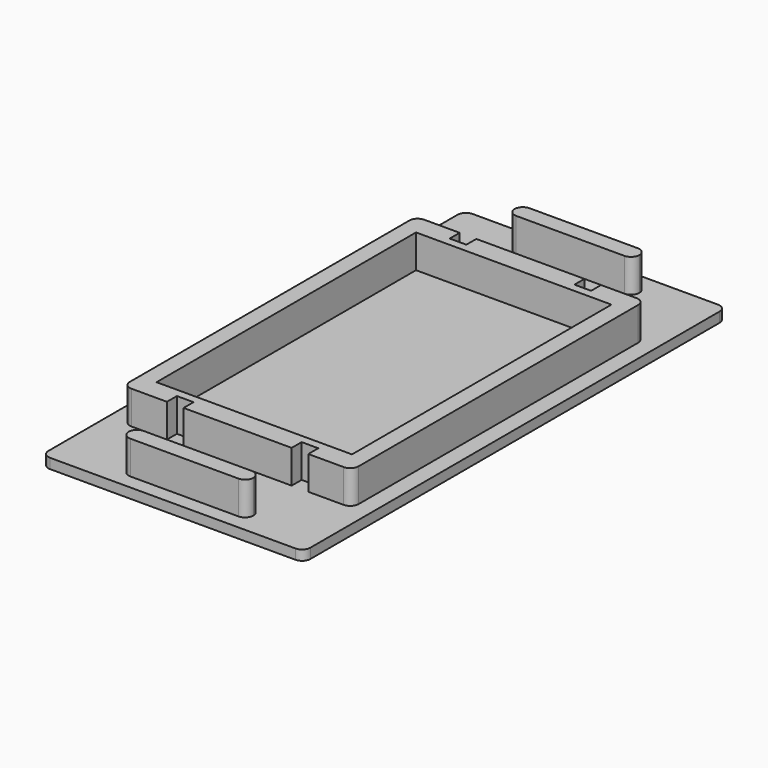
from build123d import *

# Parameters (mm, degrees)
F0_W     = 31.5
F0_H     = 63.5
F0_W_2   = 23.5
F0_H_2   = 39
F0_W_3   = 15
F0_H_3   = 2
F0_W_4   = 2
F0_H_4   = 1.5
F1_DEPTH = 1.2
F2_DEPTH = 4
F3_R     = 0.99999


# Not quite as in the source:
# - a fillet or chamfer is up to 0.001 mm smaller than in the source, because OpenCascade refuses the exact size


with BuildPart() as f1:
    # F0 (on Top) → F1 (new body)
    with BuildSketch(Plane.XY):
        Rectangle(F0_W, F0_H)
        Polygon((13.75, -22), (13.75, -30), (7.5, -30), (-7.5, -30), (-13.75, -30), (-13.75, -22), (-13.75, 22), (-13.75, 30), (-7.5, 30), (7.5, 30), (13.75, 30), (13.75, 22), align=None, mode=Mode.SUBTRACT)
        Rectangle(F0_W_2, F0_H_2)
        Polygon((-7.5, -28), (7.5, -28), (11.75, -28), (11.75, -22), (8.5, -22), (6.5, -22), (-6.5, -22), (-8.5, -22), (-11.75, -22), (-11.75, -28), align=None)
        Polygon((8.5, 22), (11.75, 22), (11.75, 28), (7.5, 28), (-7.5, 28), (-11.75, 28), (-11.75, 22), (-8.5, 22), (-6.5, 22), (6.5, 22), align=None)
        Polygon((-13.75, 22), (-13.75, -22), (-11.75, -22), (-11.75, -19.5), (-11.75, 19.5), (-11.75, 22), align=None)
        Polygon((11.75, -22), (13.75, -22), (13.75, 22), (11.75, 22), (11.75, 19.5), (11.75, -19.5), align=None)
        Polygon((8.5, -22), (11.75, -22), (11.75, -19.5), (-11.75, -19.5), (-11.75, -22), (-8.5, -22), (-8.5, -20.5), (-6.5, -20.5), (-6.5, -22), (6.5, -22), (6.5, -20.5), (8.5, -20.5), align=None)
        Polygon((11.75, 19.5), (11.75, 22), (8.5, 22), (8.5, 20.5), (6.5, 20.5), (6.5, 22), (-6.5, 22), (-6.5, 20.5), (-8.5, 20.5), (-8.5, 22), (-11.75, 22), (-11.75, 19.5), align=None)
        with Locations((0, -29)):
            Rectangle(F0_W_3, F0_H_3)
        with Locations((0, 29)):
            Rectangle(F0_W_3, F0_H_3)
        Polygon((7.5, -30), (13.75, -30), (13.75, -22), (11.75, -22), (11.75, -28), (7.5, -28), align=None)
        Polygon((-13.75, -30), (-7.5, -30), (-7.5, -28), (-11.75, -28), (-11.75, -22), (-13.75, -22), align=None)
        Polygon((11.75, 22), (13.75, 22), (13.75, 30), (7.5, 30), (7.5, 28), (11.75, 28), align=None)
        Polygon((-13.75, 30), (-13.75, 22), (-11.75, 22), (-11.75, 28), (-7.5, 28), (-7.5, 30), align=None)
        with Locations((-7.5, 21.25)):
            Rectangle(F0_W_4, F0_H_4)
        with Locations((7.5, 21.25)):
            Rectangle(F0_W_4, F0_H_4)
        with Locations((-7.5, -21.25)):
            Rectangle(F0_W_4, F0_H_4)
        with Locations((7.5, -21.25)):
            Rectangle(F0_W_4, F0_H_4)
    extrude(amount=-F1_DEPTH)

    # F0 (on Top) → F2 (join)
    with BuildSketch(Plane.XY):
        Polygon((-13.75, 22), (-13.75, -22), (-11.75, -22), (-11.75, -19.5), (-11.75, 19.5), (-11.75, 22), align=None)
        Polygon((11.75, 19.5), (11.75, 22), (8.5, 22), (8.5, 20.5), (6.5, 20.5), (6.5, 22), (-6.5, 22), (-6.5, 20.5), (-8.5, 20.5), (-8.5, 22), (-11.75, 22), (-11.75, 19.5), align=None)
        Polygon((11.75, -22), (13.75, -22), (13.75, 22), (11.75, 22), (11.75, 19.5), (11.75, -19.5), align=None)
        Polygon((8.5, -22), (11.75, -22), (11.75, -19.5), (-11.75, -19.5), (-11.75, -22), (-8.5, -22), (-8.5, -20.5), (-6.5, -20.5), (-6.5, -22), (6.5, -22), (6.5, -20.5), (8.5, -20.5), align=None)
        with Locations((0, 29)):
            Rectangle(F0_W_3, F0_H_3)
        with Locations((0, -29)):
            Rectangle(F0_W_3, F0_H_3)
    extrude(amount=F2_DEPTH)

    # F3 (radius 1 in the source; OpenCascade refuses exactly that, so slightly less here)
    f3_edges = [f1.edges().sort_by_distance(p)[0] for p in [
        (-13.75, 22, 2),
        (13.75, 22, 2),
        (13.75, -22, 2),
        (-13.75, -22, 2),
        (-15.75, -31.75, -0.6),
        (15.75, -31.75, -0.6),
        (-15.75, 31.75, -0.6),
        (15.75, 31.75, -0.6),
        (-7.5, -30, 2),
        (7.5, -30, 2),
        (7.5, -28, 2),
        (-7.5, -28, 2),
        (-7.5, 28, 2),
        (7.5, 28, 2),
        (7.5, 30, 2),
        (-7.5, 30, 2),
    ]]
    fillet(f3_edges, radius=F3_R)


solid = f1.part
